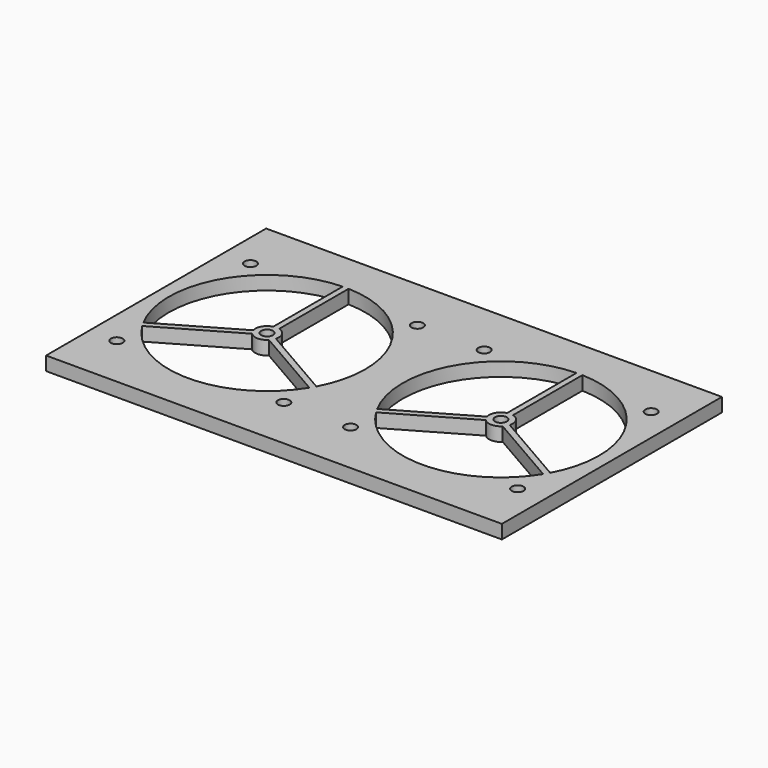
from build123d import *

# Parameters (mm, degrees)
F0_W     = 116
F0_H     = 70
F0_R     = 1.5
F1_DEPTH = 3.5
F2_D     = 3


# Not quite as in the source:
# - a feature names something its author has since deleted; it is built from what else it names


with BuildPart() as f1:
    # F0 (on Top) → F1 (new body)
    with BuildSketch(Plane.XY):
        Rectangle(F0_W, F0_H)
        with BuildLine():
            ThreePointArc((-8.4841098843, -13.1438927866), (-29.75, -25), (-51.0158901157, -13.1438927866))
            Line((-51.0158901157, -13.1438927866), (-31.8905764747, -2.1018878077))
            ThreePointArc((-31.8905764747, -2.1018878077), (-29.75, -3), (-27.6094235253, -2.1018878077))
            Line((-27.6094235253, -2.1018878077), (-8.4841098843, -13.1438927866))
        make_face(mode=Mode.SUBTRACT)
        with BuildLine():
            Line((31.8905764747, -2.1018878077), (51.0158901157, -13.1438927866))
            ThreePointArc((51.0158901157, -13.1438927866), (29.75, -25), (8.4841098843, -13.1438927866))
            Line((8.4841098843, -13.1438927866), (27.6094235253, -2.1018878077))
            ThreePointArc((27.6094235253, -2.1018878077), (29.75, -3), (31.8905764747, -2.1018878077))
        make_face(mode=Mode.SUBTRACT)
        with Locations((-29.75, 0)):
            Circle(F0_R, mode=Mode.SUBTRACT)
        with BuildLine():
            ThreePointArc((-51.7658901157, -11.844854681), (-51.4006350946, 12.5), (-30.5, 24.9887474676))
            Line((-30.5, 24.9887474676), (-30.5, 2.9047375097))
            ThreePointArc((-30.5, 2.9047375097), (-32.3480762114, 1.5), (-32.6405764747, -0.802849702))
            Line((-32.6405764747, -0.802849702), (-51.7658901157, -11.844854681))
        make_face(mode=Mode.SUBTRACT)
        with BuildLine():
            Line((-29, 2.9047375097), (-29, 24.9887474676))
            ThreePointArc((-29, 24.9887474676), (-8.0993649054, 12.5), (-7.7341098843, -11.844854681))
            Line((-7.7341098843, -11.844854681), (-26.8594235253, -0.802849702))
            ThreePointArc((-26.8594235253, -0.802849702), (-27.1519237886, 1.5), (-29, 2.9047375097))
        make_face(mode=Mode.SUBTRACT)
        with BuildLine():
            ThreePointArc((7.7341098843, -11.844854681), (8.0993649054, 12.5), (29, 24.9887474676))
            Line((29, 24.9887474676), (29, 2.9047375097))
            ThreePointArc((29, 2.9047375097), (27.1519237886, 1.5), (26.8594235253, -0.802849702))
            Line((26.8594235253, -0.802849702), (7.7341098843, -11.844854681))
        make_face(mode=Mode.SUBTRACT)
        with Locations((29.75, 0)):
            Circle(F0_R, mode=Mode.SUBTRACT)
        with BuildLine():
            Line((30.5, 2.9047375097), (30.5, 24.9887474676))
            ThreePointArc((30.5, 24.9887474676), (51.4006350946, 12.5), (51.7658901157, -11.844854681))
            Line((51.7658901157, -11.844854681), (32.6405764747, -0.802849702))
            ThreePointArc((32.6405764747, -0.802849702), (32.3480762114, 1.5), (30.5, 2.9047375097))
        make_face(mode=Mode.SUBTRACT)
    extrude(amount=F1_DEPTH)

    # F2 (through all)
    with Locations(Plane(origin=(0, 0, 0), x_dir=(1, 0, 0), z_dir=(0, 0, -1))):
        with Locations((-51, -21.25), (-51, 21.25), (-8.5, 21.25), (-8.5, -21.25), (8.5, -21.25), (8.5, 21.25), (51, 21.25), (51, -21.25)):
            Hole(F2_D / 2)


solid = f1.part
